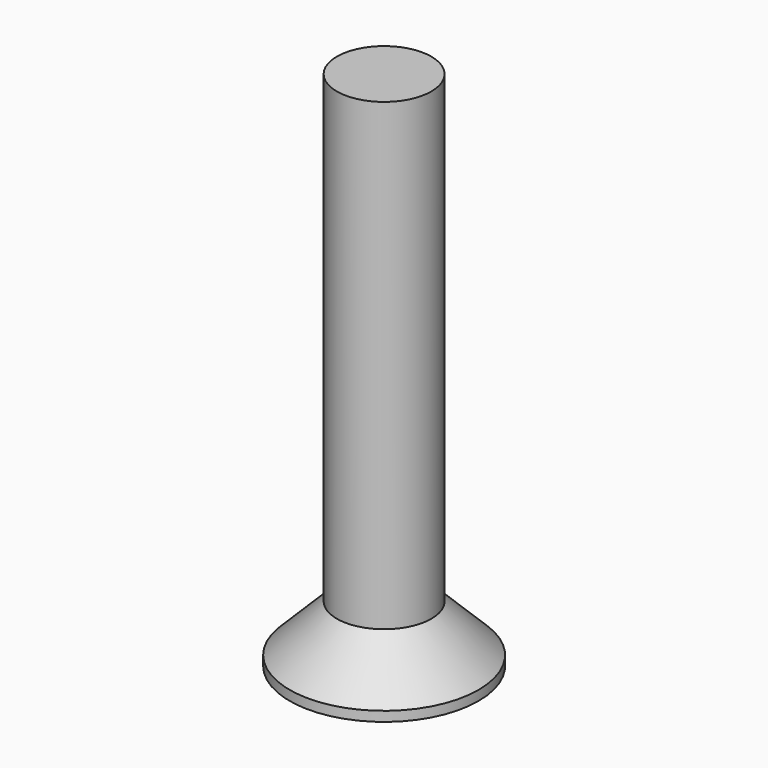
from build123d import *

# Parameters (mm, degrees)
F0_R        = 1.45
F1_DEPTH    = 14.2
F2_R        = 2.9
F3_DEPTH    = 1.8
F4_W        = 1
F4_H        = 1
F5_DEPTH    = 1.5
F6_S5_R     = 1.45
F6_T6_DEPTH = 6


# Not quite as in the source:
# - a fillet or chamfer that OpenCascade refuses, or shapes differently, is made with other operations: its cross-section is extruded or revolved along the edge and cut away or added


with BuildPart() as f1:
    # F0 (on Top) → F1 (new body)
    with BuildSketch(Plane.XY):
        Circle(F0_R)
    extrude(amount=F1_DEPTH)

    # F2 (on Top) → F3 (join)
    with BuildSketch(Plane.XY):
        Circle(F2_R)
    extrude(amount=-F3_DEPTH)

    # F4 (on face) → F5 (cut)
    with BuildSketch(Plane(origin=(0, 0, -1.8), x_dir=(1, 0, 0), z_dir=(0, 0, -1))):
        with Locations((1, 0)):
            Rectangle(F4_W, F4_H)
        Rectangle(F4_W, F4_H)
        with Locations((0, 1)):
            Rectangle(F4_W, F4_H)
        with Locations((-1, 0)):
            Rectangle(F4_W, F4_H)
        with Locations((0, -1)):
            Rectangle(F4_W, F4_H)
    extrude(amount=-F5_DEPTH, mode=Mode.SUBTRACT)

    # F6: chamfer of 1.5 on 1 edges, made by hand


with BuildPart() as f6_tool2:
    # F6_s3 → F6_t4 (revolve)
    with BuildSketch(Plane.XZ):
        Polygon((2.9, -1.5), (1.4, 0), (2.9, 0), align=None)
    revolve(axis=Axis((0, 0, 0), (0, 0, 1)))

    # F6_s5 → F6_t6 (cut, symmetric)
    with BuildSketch(Plane.XY.offset(-0.7)):
        Circle(F6_S5_R)
    extrude(amount=F6_T6_DEPTH, both=True, mode=Mode.SUBTRACT)


with BuildPart() as f1_1:
    add(f1.part)

    # F6_t1: cut F6_tool2
    add(f6_tool2.part, mode=Mode.SUBTRACT)


solid = f1_1.part
